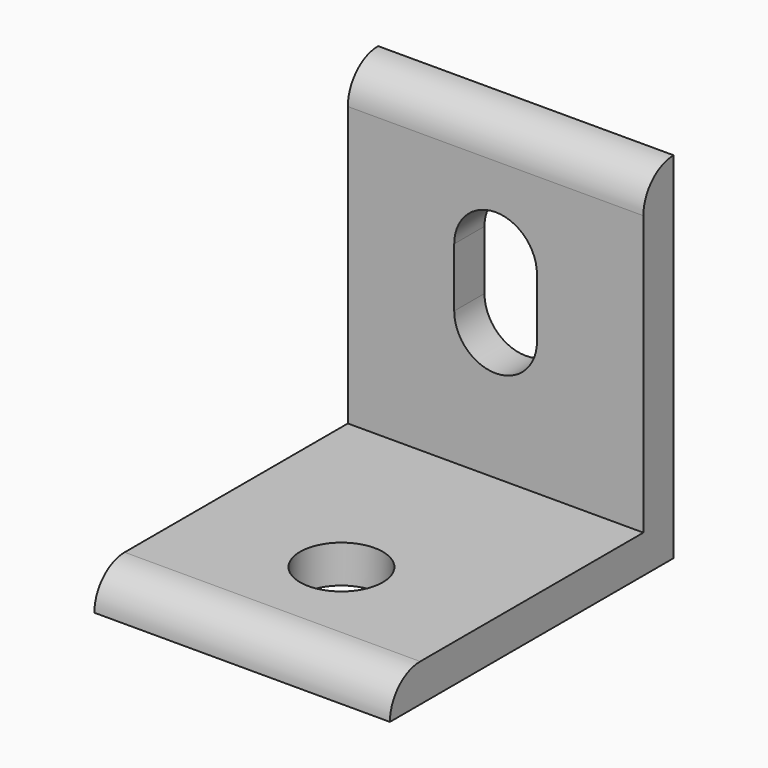
from build123d import *

# Parameters (mm, degrees)
F0_W     = 25
F0_H     = 26.8
F0_R     = 3.5
F1_DEPTH = 3.2
F0_H_2   = 3.2
F2_DEPTH = 30
F4_DEPTH = 3.2
F5_R     = 3.19999
F6_R     = 3.19999


# Not quite as in the source:
# - a fillet or chamfer is up to 0.001 mm smaller than in the source, because OpenCascade refuses the exact size


with BuildPart() as f1:
    # F0 (on Top) → F1 (new body)
    with BuildSketch(Plane.XY):
        with Locations((0, -1.6)):
            Rectangle(F0_W, F0_H)
        with Locations((0, -4.5)):
            Circle(F0_R, mode=Mode.SUBTRACT)
    extrude(amount=F1_DEPTH)

    # F0 (on Top) → F2 (join)
    with BuildSketch(Plane.XY):
        with Locations((0, 13.4)):
            Rectangle(F0_W, F0_H_2)
    extrude(amount=F2_DEPTH)

    # F3 (on face) → F4 (cut)
    with BuildSketch(Plane(origin=(0, 15, 0), x_dir=(-1, 0, 0), z_dir=(0, 1, 0))):
        with BuildLine():
            Line((-3.5, 19.5), (-3.5, 14.5))
            ThreePointArc((-3.5, 14.5), (0, 11), (3.5, 14.5))
            Line((3.5, 14.5), (3.5, 19.5))
            ThreePointArc((3.5, 19.5), (0, 23), (-3.5, 19.5))
        make_face()
    extrude(amount=-F4_DEPTH, mode=Mode.SUBTRACT)

    # F5 (radius 3.2 in the source; OpenCascade refuses exactly that, so slightly less here)
    f5_edges = [f1.edges().sort_by_distance(p)[0] for p in [
        (0, 11.8, 30),
    ]]
    fillet(f5_edges, radius=F5_R)

    # F6 (radius 3.2 in the source; OpenCascade refuses exactly that, so slightly less here)
    f6_edges = [f1.edges().sort_by_distance(p)[0] for p in [
        (0, -15, 3.2),
    ]]
    fillet(f6_edges, radius=F6_R)


solid = f1.part
